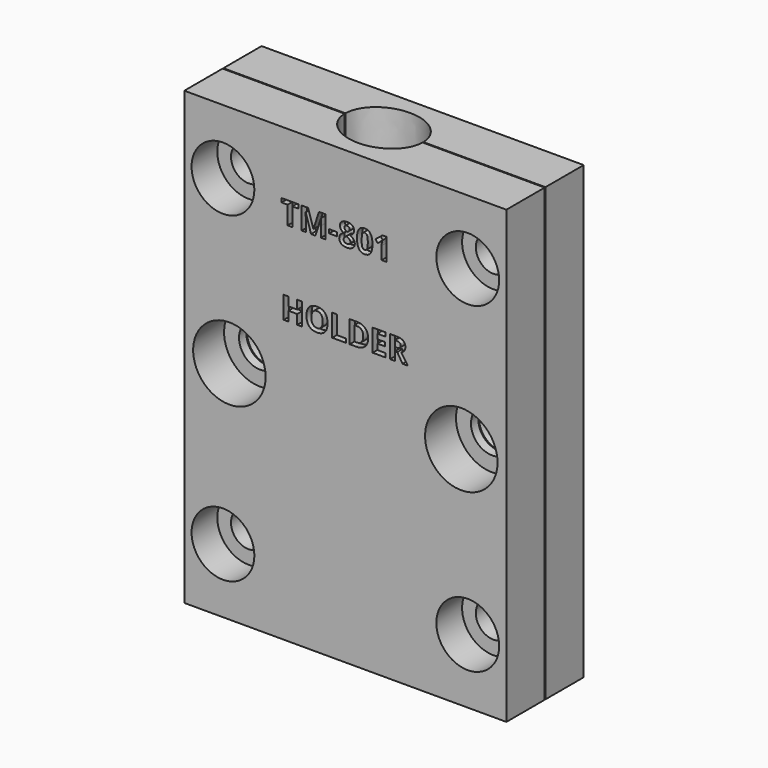
from build123d import *

# Parameters (mm, degrees)
F2_W            = 50
F2_H            = 15
F3_DEPTH        = 35
F4_DEPTH        = 35.001
F5_DEPTH        = 25
F7_D            = 5.5
F7_CBORE_D      = 9.75
F7_CBORE_DEPTH  = 5
F8_R            = 2.75
F9_DEPTH        = 5
F10_DEPTH       = 5
F13_D           = 6.6
F13_CBORE_D     = 11.25
F13_CBORE_DEPTH = 6
F15_DEPTH       = 70.0010001
F16_TEXT_SIZE   = 4.8176446234
F17_DEPTH       = 1
F18_TEXT_SIZE   = 6.0220557793
F19_DEPTH       = 1


# Not quite as in the source:
# - Text() gives the source's letters only with a copy of the font that has no kerning and outlines rounded to 1/6400 em; it was checked with that copy


with BuildPart() as f3:
    # F2 (on Top) → F3 (new body)
    with BuildSketch(Plane.XY):
        Rectangle(F2_W, F2_H)
    extrude(amount=-F3_DEPTH)

    # F1 (on face) → F4 (cut, through all)
    with BuildSketch(Plane.XY):
        with BuildLine():
            add(Edge.make_bspline(
                [(-6.05, 0), (-6.05, -8.7468565782), (3.025, -4.3734282891), (12.1, 0), (3.025, 4.3734282891), (-6.05, 8.7468565782), (-6.05, 0)],
                knots=[0, 0, 0, 2.0943951024, 2.0943951024, 4.1887902048, 4.1887902048, 6.2831853072, 6.2831853072, 6.2831853072], degree=2, weights=[1, 0.5, 1, 0.5, 1, 0.5, 1]))
        make_face()
    extrude(amount=-F4_DEPTH, mode=Mode.SUBTRACT)

    # F0 (on Top) → F5 (cut)
    with BuildSketch(Plane.XY):
        with BuildLine():
            add(Edge.make_bspline(
                [(-10.05, 0), (-10.05, -10.4789073858), (5.025, -5.2394536929), (20.1, 0), (5.025, 5.2394536929), (-10.05, 10.4789073858), (-10.05, 0)],
                knots=[0, 0, 0, 2.0943951024, 2.0943951024, 4.1887902048, 4.1887902048, 6.2831853072, 6.2831853072, 6.2831853072], degree=2, weights=[1, 0.5, 1, 0.5, 1, 0.5, 1]))
        make_face()
    extrude(amount=-F5_DEPTH, mode=Mode.SUBTRACT)

    # F7 (through all)
    with Locations(Plane.XZ.offset(7.5)):
        with Locations((-19, -25), (19, -25)):
            CounterBoreHole(F7_D / 2, F7_CBORE_D / 2, F7_CBORE_DEPTH)

    # F8 (on face) → F9 (cut)
    with BuildSketch(Plane(origin=(0, 7.5, 0), x_dir=(-1, 0, 0), z_dir=(0, 1, 0))):
        Polygon((-21.3382685902, -29.05), (-16.6617314098, -29.05), (-14.3234628196, -25), (-16.6617314098, -20.95), (-21.3382685902, -20.95), (-23.6765371804, -25), align=None)
        with Locations((-19, -25)):
            Circle(F8_R, mode=Mode.SUBTRACT)
    extrude(amount=-F9_DEPTH, mode=Mode.SUBTRACT)

    # F8 (on face) → F10 (cut)
    with BuildSketch(Plane(origin=(0, 7.5, 0), x_dir=(-1, 0, 0), z_dir=(0, 1, 0))):
        Polygon((-21.3382685902, -29.05), (-16.6617314098, -29.05), (-14.3234628196, -25), (-16.6617314098, -20.95), (-21.3382685902, -20.95), (-23.6765371804, -25), align=None)
        Polygon((14.3234628196, -25), (16.6617314098, -29.05), (21.3382685902, -29.05), (23.6765371804, -25), (21.3382685902, -20.95), (16.6617314098, -20.95), align=None)
    extrude(amount=-F10_DEPTH, mode=Mode.SUBTRACT)

    # F11: F3 across face


with BuildPart() as f3_1:
    add(f3.part)
    add(f3.part.mirror(Plane.XY))

    # F13 (through all)
    with Locations(Plane.XZ.offset(7.5)):
        with Locations((-18, 0), (18, 0)):
            CounterBoreHole(F13_D / 2, F13_CBORE_D / 2, F13_CBORE_DEPTH)

    # F14 (on face) → F15 (cut, through all)
    with BuildSketch(Plane.XY.offset(35)):
        with BuildLine():
            Line((-25, 0.075), (-25, -0.075))
            Line((-25, -0.075), (-6.0493328093, -0.075))
            add(Edge.make_bspline(
                [(-6.0493328093, -0.075), (-6.0495552759, -0.0624977359), (-6.0497332179, -0.0499960736), (-6.0498666461, -0.0374952401), (-6.0499555742, -0.0249954634), (-6.050000019, -0.0124969731), (-6.05, 0)],
                knots=[0.9977865937, 0.9977865937, 0.9977865937, 0.9977865937, 0.9977865937, 0.9977865937, 0.9977865937, 1, 1, 1, 1, 1, 1, 1], degree=6))
            add(Edge.make_bspline(
                [(-6.05, 0), (-6.050000019, 0.0124969731), (-6.0499555742, 0.0249954634), (-6.0498666461, 0.0374952401), (-6.0497332179, 0.0499960736), (-6.0495552759, 0.0624977359), (-6.0493328093, 0.075)],
                knots=[0, 0, 0, 0, 0, 0, 0, 0.0021662456, 0.0021662456, 0.0021662456, 0.0021662456, 0.0021662456, 0.0021662456, 0.0021662456], degree=6))
            Line((-6.0493328093, 0.075), (-25, 0.075))
        make_face()
        with BuildLine():
            add(Edge.make_bspline(
                [(6.0493329011, 0.075), (6.0495553154, 0.0625011784), (6.0497332541, 0.0500016078), (6.0498667103, 0.0375014933), (6.0499556795, 0.0250010408), (6.0500001594, 0.0125004571), (6.0500001411, -0.0125006489), (6.0499556465, -0.0250012746), (6.0498666664, -0.0375017246), (6.0497332029, -0.0500017965), (6.0495552604, -0.0625012887), (6.0493328458, -0.075)],
                knots=[0.4940793008, 0.4940793008, 0.4940793008, 0.4940793008, 0.4940793008, 0.4940793008, 0.4940793008, 0.4961842071, 0.4961842071, 0.4961842071, 0.4961842071, 0.4961842071, 0.4982891288, 0.4982891288, 0.4982891288, 0.4982891288, 0.4982891288, 0.4982891288, 0.4982891288], degree=6))
            Line((6.0493328458, -0.075), (25, -0.075))
            Line((25, -0.075), (25, 0.075))
            Line((25, 0.075), (6.0493329011, 0.075))
        make_face()
    extrude(amount=-F15_DEPTH, mode=Mode.SUBTRACT)

    # F16 (on face) → F17 (cut)
    with BuildSketch(Plane.XZ.offset(7.5)):
        with Locations((-10, 21.8060297056)):
            Text('TM-801', F16_TEXT_SIZE, font='Open Sans', font_style=FontStyle.BOLD, text_align=(TextAlign.LEFT, TextAlign.BOTTOM))
        with Locations((-10, 8.7020363298)):
            Text('HOLDER', F16_TEXT_SIZE, font='Open Sans', font_style=FontStyle.BOLD, text_align=(TextAlign.LEFT, TextAlign.BOTTOM))
    extrude(amount=-F17_DEPTH, mode=Mode.SUBTRACT)

    # F18 (on face) → F19 (cut)
    with BuildSketch(Plane(origin=(0, 7.5, 0), x_dir=(-1, 0, 0), z_dir=(0, 1, 0))):
        with Locations((-12.5, -4.3358801611)):
            Text('TM-801', F18_TEXT_SIZE, font='Open Sans', font_style=FontStyle.BOLD, text_align=(TextAlign.LEFT, TextAlign.BOTTOM))
        with Locations((-12.5, -12.5258760209)):
            Text('HOLDER', F18_TEXT_SIZE, font='Open Sans', font_style=FontStyle.BOLD, text_align=(TextAlign.LEFT, TextAlign.BOTTOM))
    extrude(amount=-F19_DEPTH, mode=Mode.SUBTRACT)


solid = f3_1.part
